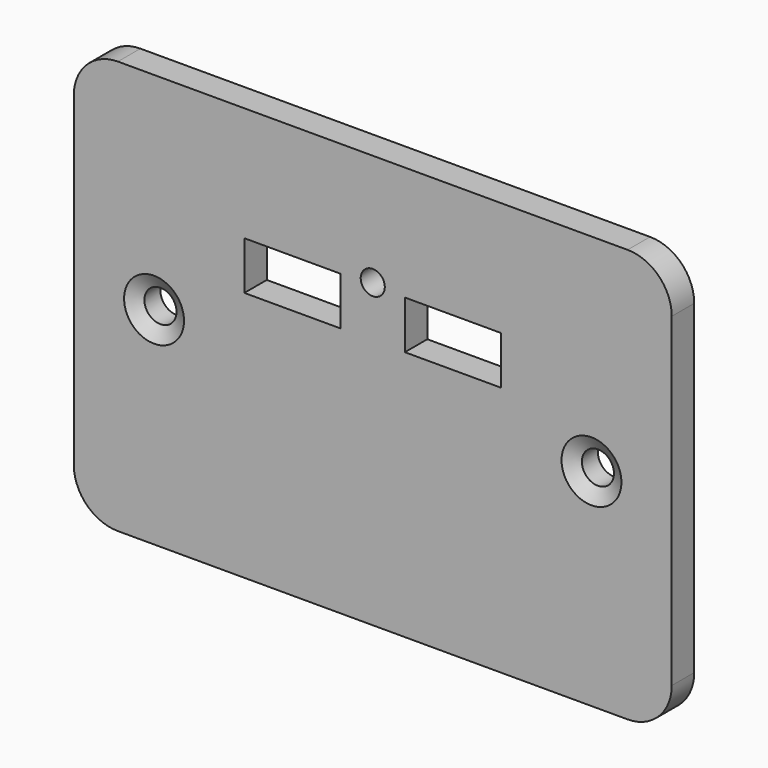
from build123d import *

# Parameters (mm, degrees)
F0_W        = 94.615
F0_H        = 65.405
F0_W_2      = 86.9950006521
F0_H_2      = 57.7850006521
F0_R        = 5.08
F0_R_2      = 2.413
F0_W_3      = 15.24
F0_H_3      = 7.62
F0_R_3      = 1.905
F0_R_4      = 2.54
F0_R_5      = 1.143
F0_W_4      = 7.112
F0_H_4      = 1.016
F1_DEPTH    = 4.445
F2_R        = 6.985
F3_SIZE2    = 2.1997045256
F3_SIZE     = 1.27
F3_2_SIZE2  = 2.1997045256
F3_2_SIZE   = 1.27
F4_T        = 2.54
F4_T3_DEPTH = 9.525


# Not quite as in the source:
# - a shell that OpenCascade refuses in one call is made with other operations: the cavity is built on its own and cut out


with BuildPart() as f1:
    # F0 (on Front) → F1 (new body)
    with BuildSketch(Plane.XZ):
        Rectangle(F0_W, F0_H)
        Rectangle(F0_W_2, F0_H_2, mode=Mode.SUBTRACT)
        Rectangle(F0_W_2, F0_H_2)
        with Locations((-34.6075, 0)):
            Circle(F0_R, mode=Mode.SUBTRACT)
        Polygon((24.765, 23.495), (24.765, -23.495), (3.556, -23.495), (-3.556, -23.495), (-24.765, -23.495), (-24.765, 23.495), align=None, mode=Mode.SUBTRACT)
        with Locations((34.6075, 0)):
            Circle(F0_R, mode=Mode.SUBTRACT)
        Polygon((-3.556, -22.479), (3.556, -22.479), (23.749, -22.479), (23.749, 22.479), (-23.749, 22.479), (-23.749, -22.479), align=None)
        with Locations((-19.685, -18.0975)):
            Circle(F0_R_2, mode=Mode.SUBTRACT)
        with Locations((19.685, -18.0975)):
            Circle(F0_R_2, mode=Mode.SUBTRACT)
        with Locations((-12.7, 10.795)):
            Rectangle(F0_W_3, F0_H_3, mode=Mode.SUBTRACT)
        with Locations((-19.685, 18.0975)):
            Circle(F0_R_2, mode=Mode.SUBTRACT)
        with Locations((0, 15.0338392705)):
            Circle(F0_R_3, mode=Mode.SUBTRACT)
        with Locations((12.7, 10.795)):
            Rectangle(F0_W_3, F0_H_3, mode=Mode.SUBTRACT)
        with Locations((19.685, 18.0975)):
            Circle(F0_R_2, mode=Mode.SUBTRACT)
        Polygon((3.556, -23.495), (24.765, -23.495), (24.765, 23.495), (-24.765, 23.495), (-24.765, -23.495), (-3.556, -23.495), (-3.556, -22.479), (-23.749, -22.479), (-23.749, 22.479), (23.749, 22.479), (23.749, -22.479), (3.556, -22.479), align=None)
        with Locations((34.6075, 0)):
            Circle(F0_R)
        with Locations((34.6075, 0)):
            Circle(F0_R_4, mode=Mode.SUBTRACT)
        with Locations((-34.6075, 0)):
            Circle(F0_R)
        with Locations((-34.6075, 0)):
            Circle(F0_R_4, mode=Mode.SUBTRACT)
        with Locations((-19.685, 18.0975)):
            Circle(F0_R_2)
        with Locations((-19.685, 18.0975)):
            Circle(F0_R_5, mode=Mode.SUBTRACT)
        with Locations((-19.685, -18.0975)):
            Circle(F0_R_2)
        with Locations((-19.685, -18.0975)):
            Circle(F0_R_5, mode=Mode.SUBTRACT)
        with Locations((19.685, -18.0975)):
            Circle(F0_R_2)
        with Locations((19.685, -18.0975)):
            Circle(F0_R_5, mode=Mode.SUBTRACT)
        with Locations((19.685, 18.0975)):
            Circle(F0_R_2)
        with Locations((19.685, 18.0975)):
            Circle(F0_R_5, mode=Mode.SUBTRACT)
        with Locations((0, -22.987)):
            Rectangle(F0_W_4, F0_H_4)
        with Locations((-19.685, 18.0975)):
            Circle(F0_R_5)
        with Locations((-19.685, -18.0975)):
            Circle(F0_R_5)
        with Locations((19.685, -18.0975)):
            Circle(F0_R_5)
        with Locations((19.685, 18.0975)):
            Circle(F0_R_5)
    extrude(amount=F1_DEPTH)

    # F2
    f2_edges = [f1.edges().sort_by_distance(p)[0] for p in [
        (-47.3075, -2.2225, 32.7025),
        (-47.3075, -2.2225, -32.7025),
        (47.3075, -2.2225, 32.7025),
        (47.3075, -2.2225, -32.7025),
    ]]
    fillet(f2_edges, radius=F2_R)

    # F3
    f3_edges = [f1.edges().sort_by_distance(p)[0] for p in [
        (-37.1475, -4.445, 0),
    ]]
    f3_side = f1.faces().sort_by_distance((-37.1475, -2.2225, 0))[0]
    chamfer(f3_edges, length=F3_SIZE, length2=F3_SIZE2, reference=f3_side)

    # F3#2
    f3_2_edges = [f1.edges().sort_by_distance(p)[0] for p in [
        (32.0675, -4.445, 0),
    ]]
    f3_2_side = f1.faces().sort_by_distance((32.0675, -2.2225, 0))[0]
    chamfer(f3_2_edges, length=F3_2_SIZE, length2=F3_2_SIZE2, reference=f3_2_side)

    # F4: shell of thickness 2.54, made by hand


with BuildPart() as f4_core1:
    # F4_t2: copy of F1
    add(f1.part)

    # the walls: a layer under each face that stays
    f4_faces = [f4_core1.faces().sort_by_distance(p)[0] for p in [
        (0, -4.445, 0),
        (30.9676477372, -3.81, 0),
        (-38.2473522628, -3.81, 0),
        (0, -2.2225, -32.7025),
        (-45.2616408666, -2.2225, -30.6566408666),
        (45.2616408666, -2.2225, -30.6566408666),
        (-47.3075, -2.2225, 0),
        (47.3075, -2.2225, 0),
        (-45.2616408666, -2.2225, 30.6566408666),
        (45.2616408666, -2.2225, 30.6566408666),
        (0, -2.2225, 32.7025),
        (20.32, -2.2225, 10.795),
        (12.7, -2.2225, 6.985),
        (5.08, -2.2225, 10.795),
        (12.7, -2.2225, 14.605),
        (-12.7, -2.2225, 6.985),
        (-20.32, -2.2225, 10.795),
        (-12.7, -2.2225, 14.605),
        (-5.08, -2.2225, 10.795),
        (-1.905, -2.2225, 15.0338392705),
        (32.0675, -1.5875, 0),
        (-37.1475, -1.5875, 0),
    ]]
    thicken(f4_faces, amount=-F4_T, mode=Mode.SUBTRACT)

    # F4_s4 → F4_t3 (cut)
    with BuildSketch(Plane.XZ.offset(-2.54)):
        Polygon((20.2946, 14.5796), (22.86, 14.605), (22.86, 17.145), (20.32, 17.145), align=None)
        Polygon((20.2946, 7.0104), (22.86, 6.985), (22.86, 4.445), (20.32, 4.445), align=None)
        Polygon((5.1054, 7.0104), (5.08, 4.445), (2.54, 4.445), (2.54, 6.985), align=None)
        Polygon((5.1054, 14.5796), (2.54, 14.605), (2.54, 17.145), (5.08, 17.145), align=None)
        Polygon((-5.1054, 7.0104), (-5.08, 4.445), (-2.54, 4.445), (-2.54, 6.985), align=None)
        Polygon((-20.2946, 7.0104), (-20.32, 4.445), (-22.86, 4.445), (-22.86, 6.985), align=None)
        Polygon((-20.2946, 14.5796), (-22.86, 14.605), (-22.86, 17.145), (-20.32, 17.145), align=None)
        Polygon((-5.1054, 14.5796), (-5.08, 17.145), (-2.54, 17.145), (-2.54, 14.605), align=None)
    extrude(amount=F4_T3_DEPTH, mode=Mode.SUBTRACT)


with BuildPart() as f1_1:
    add(f1.part)

    # what is left inside the walls is the cavity
    f4_cavity = [f4_core1.part.solids().sort_by_distance(p)[0] for p in [
        (0, -0.0254, -10.054167),
    ]]
    add(f4_cavity, mode=Mode.SUBTRACT)


solid = f1_1.part
